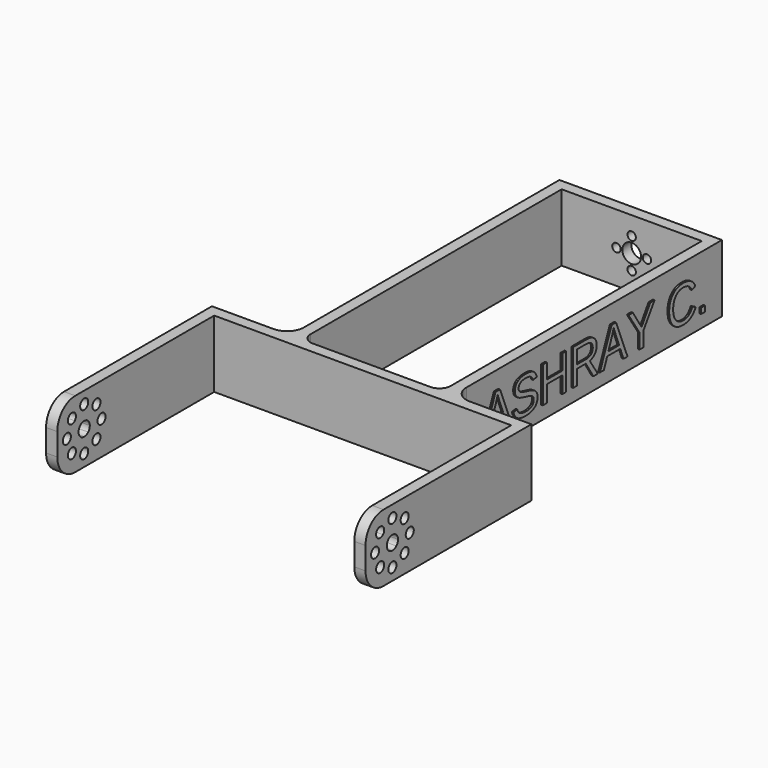
from build123d import *

# Parameters (mm, degrees)
F0_W          = 5.08
F0_H          = 152.4
F1_DEPTH      = 30.48
F2_W          = 5.08
F2_H          = 30.48
F3_DEPTH      = 66.04
F4_R          = 7.62
F5_R          = 5.08
F6_R          = 2.286
F7_DEPTH      = 254
F8_R          = 10.16
F9_TEXT_SIZE  = 23.6567902672
F11_DEPTH     = 0.762
F10_TEXT_SIZE = 23.6567902672
F12_DEPTH     = 0.762
F13_R         = 1.905
F13_R_2       = 4.2545
F14_DEPTH     = 25.4


# Not quite as in the source:
# - Text() gives the source's letters only with a copy of the font that has no kerning and outlines rounded to 1/6400 em; it was checked with that copy


with BuildPart() as f1:
    # F0 (on Top) → F1 (new body)
    with BuildSketch(Plane.XY):
        with Locations((-34.29, 78.74)):
            Rectangle(F0_W, F0_H)
        with Locations((34.29, 78.74)):
            Rectangle(F0_W, F0_H)
        Polygon((-67.31, -2.54), (67.31, -2.54), (67.31, 2.54), (36.83, 2.54), (31.75, 2.54), (-31.75, 2.54), (-36.83, 2.54), (-67.31, 2.54), align=None)
        Polygon((67.31, 2.54), (67.31, -2.54), (67.31, -91.44), (72.39, -91.44), (72.39, 2.54), align=None)
        Polygon((-67.31, -91.44), (-67.31, -2.54), (-67.31, 2.54), (-72.39, 2.54), (-72.39, -91.44), align=None)
    extrude(amount=F1_DEPTH)

    # F2 (on face) → F3 (join)
    with BuildSketch(Plane.YZ.offset(-31.75)):
        with Locations((152.4, 15.24)):
            Rectangle(F2_W, F2_H)
    extrude(amount=F3_DEPTH)

    # F4
    f4_edges = [f1.edges().sort_by_distance(p)[0] for p in [
        (-36.83, 2.54, 15.24),
        (36.83, 2.54, 15.24),
    ]]
    fillet(f4_edges, radius=F4_R)

    # F5
    f5_edges = [f1.edges().sort_by_distance(p)[0] for p in [
        (-31.75, 2.54, 15.24),
        (31.75, 2.54, 15.24),
    ]]
    fillet(f5_edges, radius=F5_R)

    # F6 (on face) → F7 (cut)
    with BuildSketch(Plane(origin=(-72.39, 0, 0), x_dir=(0, -1, 0), z_dir=(-1, 0, 0))):
        with BuildLine():
            ThreePointArc((85.4367182377, 22.1907182377), (82.2759039113, 24.302706849), (81.5342721359, 20.5742721359))
            ThreePointArc((81.5342721359, 20.5742721359), (84.0255325641, 20.0787296264), (85.4367182377, 22.1907182377))
        make_face()
        with BuildLine():
            ThreePointArc((78.486, 25.0698), (74.5835538982, 26.6862461018), (76.2, 22.7838))
            ThreePointArc((76.2, 22.7838), (77.8164461018, 23.4533538982), (78.486, 25.0698))
        make_face()
        with BuildLine():
            ThreePointArc((71.5352817623, 22.1907182377), (67.137293151, 23.0655325641), (70.8657278641, 20.5742721359))
            ThreePointArc((70.8657278641, 20.5742721359), (71.3612703736, 21.3159039113), (71.5352817623, 22.1907182377))
        make_face()
        with Locations((66.3702, 15.24)):
            Circle(F6_R)
        with BuildLine():
            ThreePointArc((71.5352817623, 8.2892817623), (71.3612703736, 9.1640960887), (70.8657278641, 9.9057278641))
            ThreePointArc((70.8657278641, 9.9057278641), (67.137293151, 7.4144674359), (71.5352817623, 8.2892817623))
        make_face()
        with BuildLine():
            ThreePointArc((78.486, 5.4102), (77.8164461018, 7.0266461018), (76.2, 7.6962))
            ThreePointArc((76.2, 7.6962), (74.5835538982, 3.7937538982), (78.486, 5.4102))
        make_face()
        with BuildLine():
            ThreePointArc((85.4367182377, 8.2892817623), (84.0255325641, 10.4012703736), (81.5342721359, 9.9057278641))
            ThreePointArc((81.5342721359, 9.9057278641), (82.2759039113, 6.177293151), (85.4367182377, 8.2892817623))
        make_face()
        with BuildLine():
            ThreePointArc((88.3158, 15.24), (86.0298, 17.526), (83.7438, 15.24))
            ThreePointArc((83.7438, 15.24), (86.0298, 12.954), (88.3158, 15.24))
        make_face()
        with BuildLine():
            Line((78.4450640303, 12.9949359697), (76.2, 15.24))
            Line((76.2, 15.24), (76.2, 12.065))
            ThreePointArc((76.2, 12.065), (77.4150198978, 12.3066824843), (78.4450640303, 12.9949359697))
        make_face()
        with BuildLine():
            Line((79.375, 15.24), (76.2, 15.24))
            Line((76.2, 15.24), (78.4450640303, 12.9949359697))
            ThreePointArc((78.4450640303, 12.9949359697), (79.1333175157, 14.0249801022), (79.375, 15.24))
        make_face()
        with BuildLine():
            Line((78.4450640303, 17.4850640303), (76.2, 15.24))
            Line((76.2, 15.24), (79.375, 15.24))
            ThreePointArc((79.375, 15.24), (79.1333175157, 16.4550198978), (78.4450640303, 17.4850640303))
        make_face()
        with BuildLine():
            Line((76.2, 18.415), (76.2, 15.24))
            Line((76.2, 15.24), (78.4450640303, 17.4850640303))
            ThreePointArc((78.4450640303, 17.4850640303), (77.4150198978, 18.1733175157), (76.2, 18.415))
        make_face()
        with BuildLine():
            ThreePointArc((76.2, 18.415), (74.9849801022, 18.1733175157), (73.9549359697, 17.4850640303))
            Line((73.9549359697, 17.4850640303), (76.2, 15.24))
            Line((76.2, 15.24), (76.2, 18.415))
        make_face()
        with BuildLine():
            ThreePointArc((73.9549359697, 17.4850640303), (73.2666824843, 16.4550198978), (73.025, 15.24))
            Line((73.025, 15.24), (76.2, 15.24))
            Line((76.2, 15.24), (73.9549359697, 17.4850640303))
        make_face()
        with BuildLine():
            Line((76.2, 15.24), (73.025, 15.24))
            ThreePointArc((73.025, 15.24), (73.2666824843, 14.0249801022), (73.9549359697, 12.9949359697))
            Line((73.9549359697, 12.9949359697), (76.2, 15.24))
        make_face()
        with BuildLine():
            Line((76.2, 15.24), (73.9549359697, 12.9949359697))
            ThreePointArc((73.9549359697, 12.9949359697), (74.9849801022, 12.3066824843), (76.2, 12.065))
            Line((76.2, 12.065), (76.2, 15.24))
        make_face()
    extrude(amount=-F7_DEPTH, mode=Mode.SUBTRACT)

    # F8
    f8_edges = [f1.edges().sort_by_distance(p)[0] for p in [
        (69.85, -91.44, 0),
        (69.85, -91.44, 30.48),
        (-69.85, -91.44, 0),
        (-69.85, -91.44, 30.48),
    ]]
    fillet(f8_edges, radius=F8_R)

    # F9 (on face) → F11 (join)
    with BuildSketch(Plane.YZ.offset(36.83)):
        with Locations((19.05, 6.35)):
            Text('ASHRAY C.', F9_TEXT_SIZE, font='Arimo', text_align=(TextAlign.LEFT, TextAlign.BOTTOM))
    extrude(amount=F11_DEPTH)

    # F10 (on face) → F12 (join)
    with BuildSketch(Plane(origin=(-36.83, 0, 0), x_dir=(0, -1, 0), z_dir=(-1, 0, 0))):
        with Locations((-146.05, 7.0971110076)):
            Text('ASHRAY C.', F10_TEXT_SIZE, font='Arimo', text_align=(TextAlign.LEFT, TextAlign.BOTTOM))
    extrude(amount=F12_DEPTH)

    # F13 (on face) → F14 (cut)
    with BuildSketch(Plane(origin=(0, 154.94, 0), x_dir=(-1, 0, 0), z_dir=(0, 1, 0))):
        with Locations((-6.9215, 15.24)):
            Circle(F13_R)
        with Locations((0, 15.24)):
            Circle(F13_R_2)
        with Locations((0, 22.1615)):
            Circle(F13_R)
        with Locations((6.9215, 15.24)):
            Circle(F13_R)
        with Locations((0, 8.3185)):
            Circle(F13_R)
    extrude(amount=-F14_DEPTH, mode=Mode.SUBTRACT)


solid = f1.part
